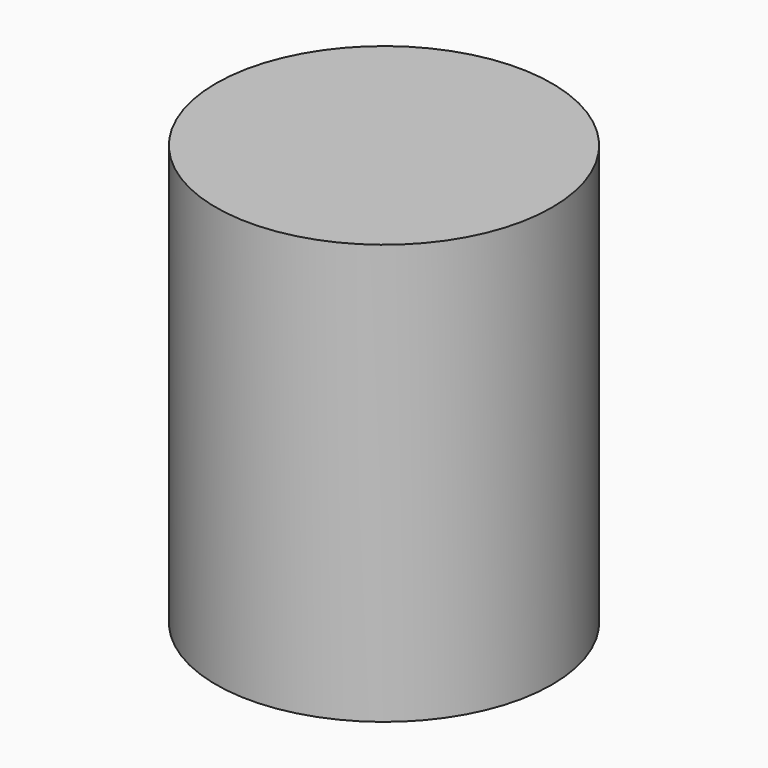
from build123d import *

# Parameters (mm, degrees)
F0_R     = 12.7
F1_DEPTH = 31.75


# Not quite as in the source:
# - the program builds the solid bodies; features that only make, move or delete a surface that nothing else refers to are left out


with BuildPart() as f1:
    # F0 (on Top) → F1 (new body)
    with BuildSketch(Plane.XY):
        Circle(F0_R)
    extrude(amount=F1_DEPTH)


solid = f1.part
